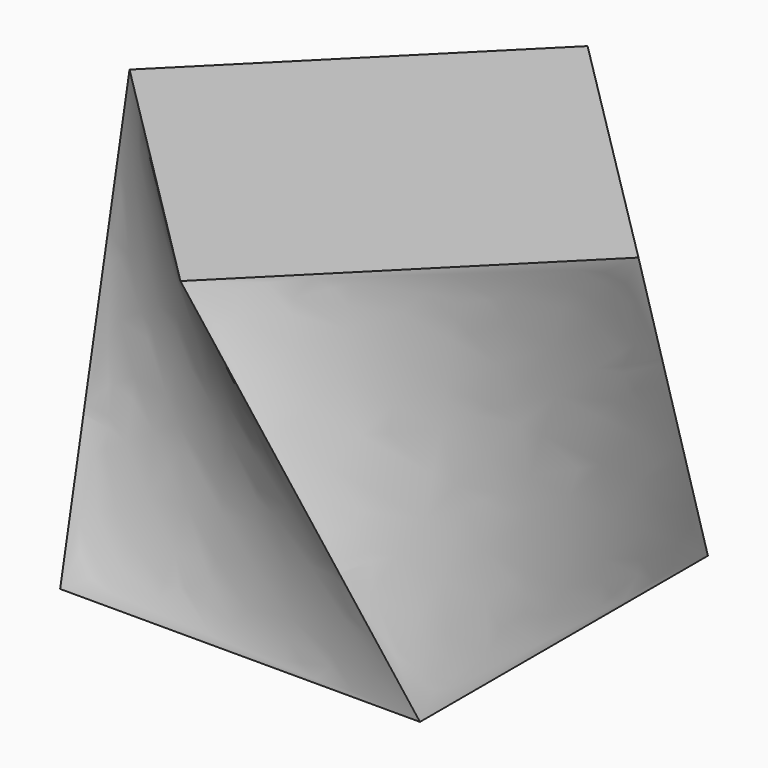
from build123d import *

# Parameters (mm, degrees)
F1_W = 25.4
F1_H = 25.4


# Not quite as in the source:
# - a variable given as a bare number and used for a length is read in inches; the dataset says mm whatever the document's units were


with BuildPart() as f4:
    # F1 (on Top) → F4 section 0
    with BuildSketch(Plane.XY):
        Rectangle(F1_W, F1_H)
    # F3 (on offset) → F4 section 1
    with BuildSketch(Plane.XY.offset(25.4)):
        Polygon((17.9605122421, 0), (0, 17.9605122421), (-17.9605122421, 0), (0, -17.9605122421), align=None)
    loft()


solid = f4.part
